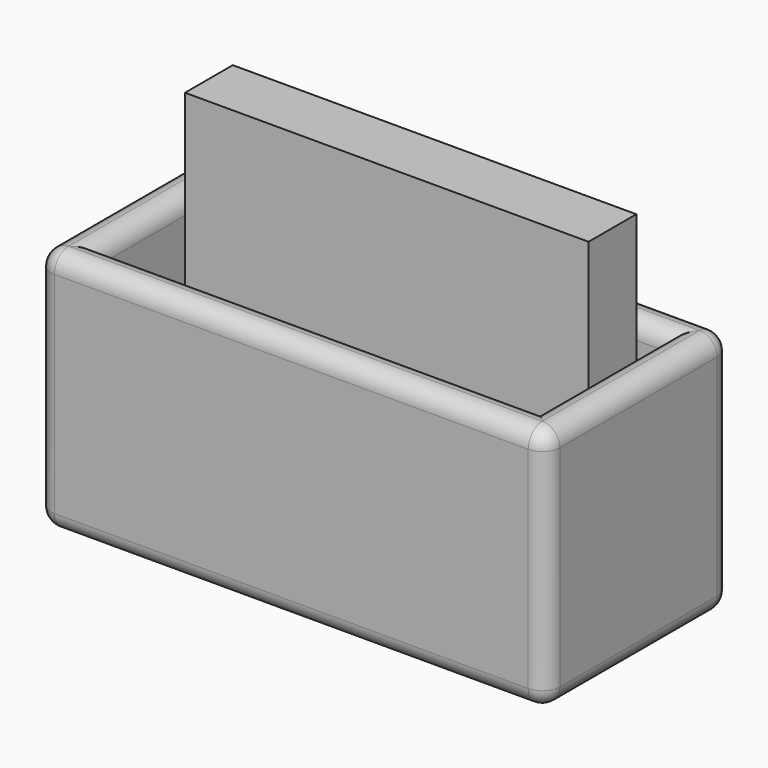
from build123d import *

# Parameters (mm, degrees)
F0_W     = 14.5
F0_H     = 6.6
F0_W_2   = 12.5
F0_H_2   = 4.6
F1_DEPTH = 7
F0_W_3   = 11.5
F0_H_3   = 1.7
F2_DEPTH = 2
F3_DEPTH = 10
F5_DEPTH = 0.4
F6_R     = 0.49999


# Not quite as in the source:
# - a fillet or chamfer is up to 0.001 mm smaller than in the source, because OpenCascade refuses the exact size


with BuildPart() as f1:
    # F0 (on Top) → F1 (new body)
    with BuildSketch(Plane.XY):
        with Locations((0.6113282288, 0)):
            Rectangle(F0_W, F0_H)
        with Locations((0.6113282288, 0)):
            Rectangle(F0_W_2, F0_H_2, mode=Mode.SUBTRACT)
    extrude(amount=F1_DEPTH)

    # F0 (on Top) → F2 (join)
    with BuildSketch(Plane.XY):
        with Locations((0.6113282288, 0)):
            Rectangle(F0_W_2, F0_H_2)
        with Locations((0.6113282288, 0.95)):
            Rectangle(F0_W_3, F0_H_3, mode=Mode.SUBTRACT)
        with Locations((0.6113282288, 0.95)):
            Rectangle(F0_W_3, F0_H_3)
    extrude(amount=F2_DEPTH)

    # F0 (on Top) → F3 (join)
    with BuildSketch(Plane.XY):
        with Locations((0.6113282288, 0.95)):
            Rectangle(F0_W_3, F0_H_3)
    extrude(amount=F3_DEPTH)

    # F4 (on face) → F5 (cut)
    with BuildSketch(Plane(origin=(0, 3.3, 0), x_dir=(-1, 0, 0), z_dir=(0, 1, 0))):
        with BuildLine():
            Line((-5.1014683965, 5.8378594238), (-5.1014683965, 6.0878594238))
            ThreePointArc((-5.1014683965, 6.0878594238), (-7.1005673821, 4.1478864664), (-5.2214683965, 2.0914626697))
            Line((-5.2214683965, 2.0914626697), (-5.2214683965, 2.3419785573))
            ThreePointArc((-5.2214683965, 2.3419785573), (-6.8504383099, 4.1478947619), (-5.1014683965, 5.8378594238))
        make_face()
        with BuildLine():
            Line((-5.2214683965, 2.3419785573), (-5.2214683965, 2.0914626697))
            ThreePointArc((-5.2214683965, 2.0914626697), (-5.0964586021, 2.0878656984), (-4.9714683965, 2.0920888959))
            Line((-4.9714683965, 2.0920888959), (-4.9714683965, 2.3426946752))
            ThreePointArc((-4.9714683965, 2.3426946752), (-5.0964555923, 2.3378666033), (-5.2214683965, 2.3419785573))
        make_face()
        with BuildLine():
            ThreePointArc((-4.9714683965, 2.0920888959), (-5.0964586021, 2.0878656984), (-5.2214683965, 2.0914626697))
            Line((-5.2214683965, 2.0914626697), (-5.2214683965, 0.5878594238))
            Line((-5.2214683965, 0.5878594238), (-4.9714683965, 0.5878594238))
            Line((-4.9714683965, 0.5878594238), (-4.9714683965, 2.0920888959))
        make_face()
        with BuildLine():
            Line((-4.9714683965, 2.3426946752), (-4.9714683965, 2.0920888959))
            ThreePointArc((-4.9714683965, 2.0920888959), (-3.6420164446, 2.7203799907), (-3.1014683965, 4.0878594238))
            Line((-3.1014683965, 4.0878594238), (-3.3514683965, 4.0878594238))
            ThreePointArc((-3.3514683965, 4.0878594238), (-3.3559614625, 3.9625376644), (-3.3694175889, 3.8378594238))
            ThreePointArc((-3.3694175889, 3.8378594238), (-3.907446743, 2.8084797729), (-4.9714683965, 2.3426946752))
        make_face()
        with BuildLine():
            Line((-5.2214683965, 4.0878594238), (-5.2214683965, 2.3419785573))
            ThreePointArc((-5.2214683965, 2.3419785573), (-5.0964555923, 2.3378666033), (-4.9714683965, 2.3426946752))
            Line((-4.9714683965, 2.3426946752), (-4.9714683965, 3.8378594238))
            Line((-4.9714683965, 3.8378594238), (-3.3694175889, 3.8378594238))
            ThreePointArc((-3.3694175889, 3.8378594238), (-3.3559614625, 3.9625376644), (-3.3514683965, 4.0878594238))
            Line((-3.3514683965, 4.0878594238), (-5.2214683965, 4.0878594238))
        make_face()
    extrude(amount=-F5_DEPTH, mode=Mode.SUBTRACT)

    # F6 (radius 0.5 in the source; OpenCascade refuses exactly that, so slightly less here)
    f6_edges = [f1.edges().sort_by_distance(p)[0] for p in [
        (7.861328, 3.3, 3.5),
        (0.611328, 3.3, 7),
        (0.611328, 3.3, 0),
        (7.861328, 0, 0),
        (7.861328, 0, 7),
        (7.861328, -3.3, 3.5),
        (0.611328, -3.3, 0),
        (-6.638672, 0, 0),
        (-6.638672, 3.3, 3.5),
        (-6.638672, -3.3, 3.5),
        (0.611328, -3.3, 7),
        (-6.638672, 0, 7),
        (0.611328, 2.3, 7),
        (0.611328, -2.3, 7),
        (-5.638672, 0, 7),
        (6.861328, 0, 7),
    ]]
    fillet(f6_edges, radius=F6_R)


solid = f1.part
